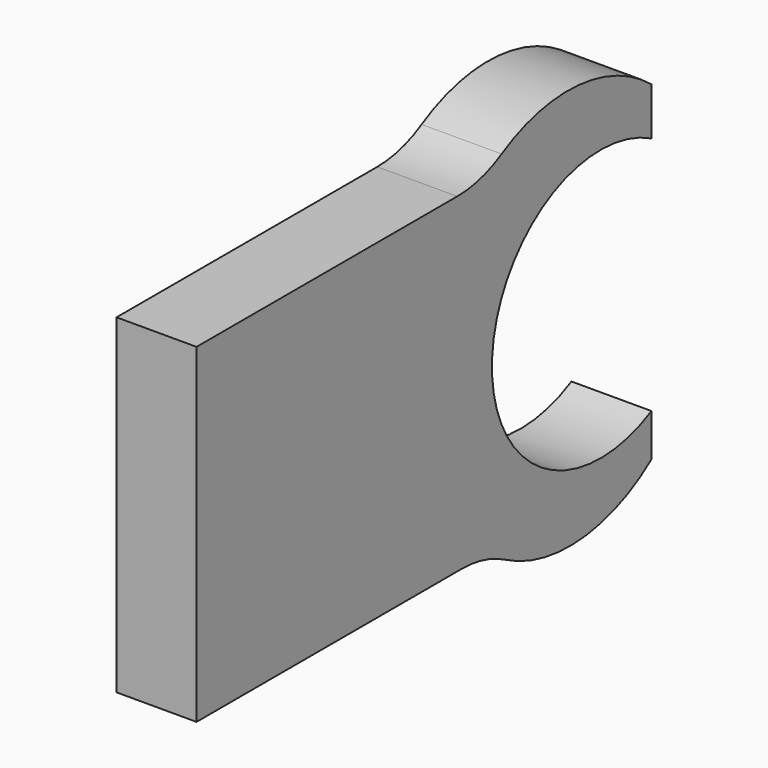
from build123d import *

# Parameters (mm, degrees)
F1_DEPTH = 3.175


# Not quite as in the source:
# - a feature names something its author has since deleted; it is built from what else it names


with BuildPart() as f1:
    # F0 (on Right) → F1 (new body)
    with BuildSketch(Plane.YZ):
        with BuildLine():
            Line((-0.0335522907, 7.0097496485), (-12.9674749849, 7.0097496485))
            Line((-12.9674749849, 7.0097496485), (-12.9674749849, -6.0952282245))
            Line((-12.9674749849, -6.0952282245), (0.1951931324, -6.0952282245))
            ThreePointArc((0.1951931324, -6.0952282245), (1.3039147966, -6.2365574954), (2.3417274082, -6.651506498))
            ThreePointArc((2.3417274082, -6.651506498), (6.055282807, -7.4637663122), (9.6017406465, -6.0952282245))
            Line((9.6017406465, -6.0952282245), (9.6017406465, -4.4064043338))
            ThreePointArc((9.6017406465, -4.4064043338), (1.6888526066, 0.3560956662), (9.6017406465, 5.1185956662))
            Line((9.6017406465, 5.1185956662), (9.6017406465, 7.0097496485))
            ThreePointArc((9.6017406465, 7.0097496485), (5.9747824086, 8.4525130692), (2.1664773001, 7.5962394284))
            ThreePointArc((2.1664773001, 7.5962394284), (1.1048786978, 7.158888427), (-0.0335522907, 7.0097496485))
        make_face()
    extrude(amount=F1_DEPTH)


solid = f1.part
